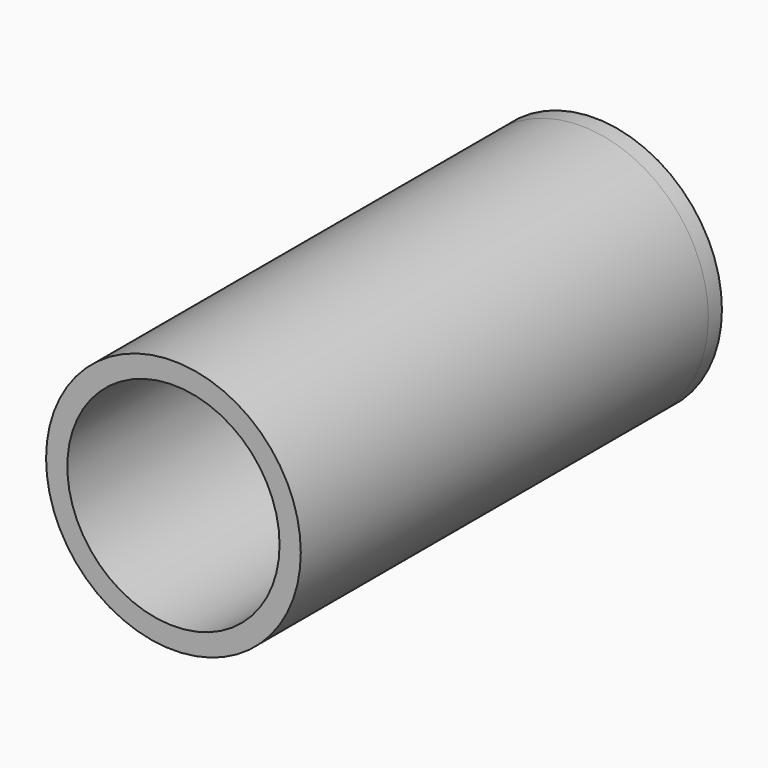
from build123d import *

# Parameters (mm, degrees)
F0_R     = 38.1
F0_R_2   = 31.75
F1_DEPTH = 152.4
F2_R     = 38.1
F2_R_2   = 31.75
F3_DEPTH = 5.08


with BuildPart() as f1:
    # F0 (on Front) → F1 (new body)
    with BuildSketch(Plane.XZ):
        Circle(F0_R)
        Circle(F0_R_2, mode=Mode.SUBTRACT)
    extrude(amount=F1_DEPTH)

    # F2 (on face) → F3 (join)
    with BuildSketch(Plane(origin=(0, 0, 0), x_dir=(-1, 0, 0), z_dir=(0, 1, 0))):
        Circle(F2_R)
        Circle(F2_R_2, mode=Mode.SUBTRACT)
        Circle(F2_R_2)
    extrude(amount=F3_DEPTH)


solid = f1.part
